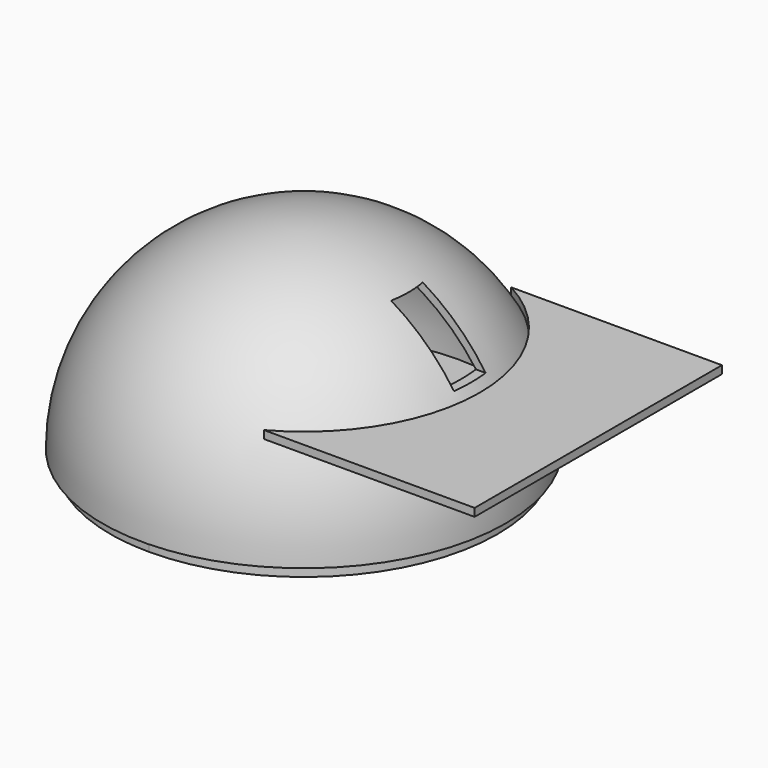
from build123d import *

# Parameters (mm, degrees)
F7_DEPTH  = 2
F10_DEPTH = 64.1
F12_DEPTH = 3
F15_W     = 5
F15_H     = 30
F16_DEPTH = 2


# Not quite as in the source:
# - the program builds the solid bodies; features that only make, move or delete a surface that nothing else refers to are left out


with BuildPart() as f1:
    # F0 (on Front) → F1 (revolve)
    with BuildSketch(Plane.XZ):
        with BuildLine():
            Line((0, 0), (51, 0))
            ThreePointArc((51, 0), (36.0624458405, 36.0624458405), (0, 51))
            Line((0, 51), (0, 0))
        make_face()
    revolve(axis=Axis((0, 0, 25.5), (0, 0, -1)))

    # F2 (on Front) → F3 (revolve, cut)
    with BuildSketch(Plane.XZ):
        with BuildLine():
            Line((0, 0), (49, 0))
            ThreePointArc((49, 0), (34.6482322781, 34.6482322781), (0, 49))
            Line((0, 49), (0, 0))
        make_face()
    revolve(axis=Axis((0, 0, 24.5), (0, 0, -1)), mode=Mode.SUBTRACT)

    # F6 (on offset) → F7 (join)
    with BuildSketch(Plane.XY.offset(25)):
        with BuildLine():
            ThreePointArc((44.452, 0), (38.1849042827, -22.757271122), (21.1507587097, -39.0976432794))
            Line((21.1507587097, -39.0976432794), (74.452, -39.0976432794))
            Line((74.452, -39.0976432794), (74.452, 0))
            Line((74.452, 0), (44.452, 0))
        make_face()
        with BuildLine():
            ThreePointArc((21.1507587097, 39.0976432794), (38.1849042827, 22.757271122), (44.452, 0))
            Line((44.452, 0), (74.452, 0))
            Line((74.452, 0), (74.452, 39.097645))
            Line((74.452, 39.097645), (21.1507587097, 39.0976432794))
        make_face()
    extrude(amount=F7_DEPTH)

    # F9 (on Right) → F10 (cut)
    with BuildSketch(Plane.YZ):
        Polygon((5, 36.0624458633), (0, 36.0624458633), (-5, 36.0624458633), (-5, 28.5624458633), (5, 28.5624458633), align=None)
        Polygon((-5, 36.0624458633), (0, 36.0624458633), (5, 36.0624458633), (5, 43.5624458633), (0, 43.5624458633), (-5, 43.5624458633), align=None)
    extrude(amount=F10_DEPTH, mode=Mode.SUBTRACT)


with BuildPart() as f12:
    # F11 (on Top) → F12 (new body)
    with BuildSketch(Plane.XY):
        with BuildLine():
            Line((-41.6476151588, 15), (-41.6476151588, 0))
            Line((-41.6476151588, 0), (-41.6476151588, -15))
            Line((-41.6476151588, -15), (-46.6476151588, -15))
            ThreePointArc((-46.6476151588, -15), (-28.8617393793, -39.5979797464), (0, -49))
            ThreePointArc((0, -49), (49, 0), (0, 49))
            ThreePointArc((0, 49), (-28.8617393793, 39.5979797464), (-46.6476151588, 15))
            Line((-46.6476151588, 15), (-41.6476151588, 15))
        make_face()
    extrude(amount=-F12_DEPTH)


with BuildPart() as f12b:
    # F11 (on Top) → F12, piece 2 (new body)
    with BuildSketch(Plane.XY):
        with BuildLine():
            Line((-46.6476151588, -15), (-46.6476151588, 0))
            Line((-46.6476151588, 0), (-49, 0))
            ThreePointArc((-49, 0), (-48.408331632, -7.591668368), (-46.6476151588, -15))
        make_face()
        with BuildLine():
            Line((-49, 0), (-46.6476151588, 0))
            Line((-46.6476151588, 0), (-46.6476151588, 15))
            ThreePointArc((-46.6476151588, 15), (-48.408331632, 7.591668368), (-49, 0))
        make_face()
    extrude(amount=-F12_DEPTH)


with BuildPart() as f16:
    # F15 (on offset) → F16 (new body)
    with BuildSketch(Plane.XY.offset(-10)):
        with Locations((-44.1476151588, 0)):
            Rectangle(F15_W, F15_H)
    extrude(amount=-F16_DEPTH)


solid = Compound([f1.part, f12.part, f12b.part, f16.part])
